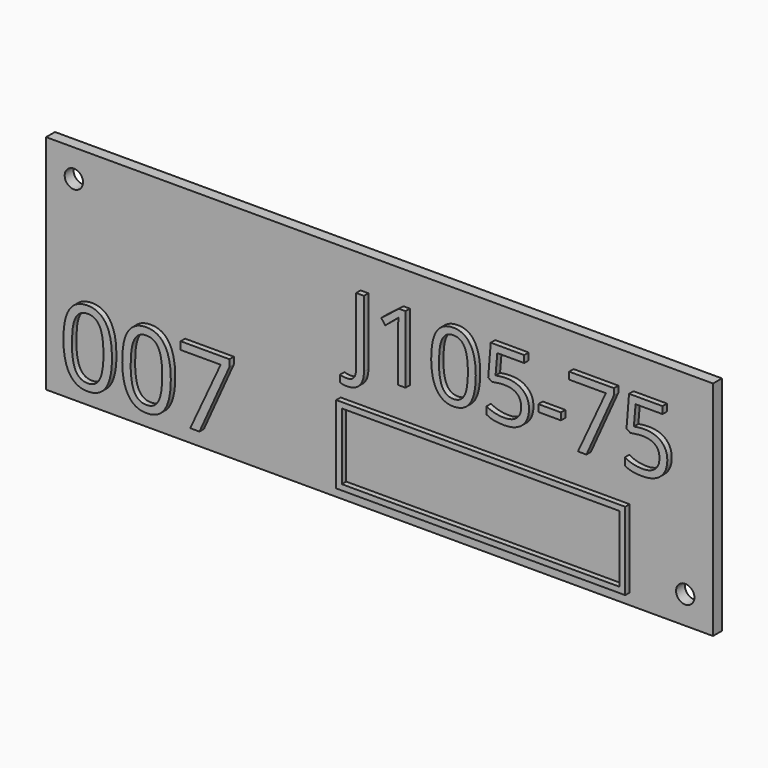
from build123d import *

# Parameters (mm, degrees)
F0_W         = 120
F0_H         = 40
F1_DEPTH     = 2
F3_D         = 3.3
F4_TEXT_SIZE = 16.9836355595
F5_DEPTH     = 1
F6_TEXT_SIZE = 18.5054667028
F7_DEPTH     = 1
F8_W         = 52
F8_H         = 14
F8_W_2       = 49.99999962
F8_H_2       = 11.99999962
F9_DEPTH     = 1


# Not quite as in the source:
# - Text() gives the source's letters only with a copy of the font that has no kerning and outlines rounded to 1/6400 em; it was checked with that copy


with BuildPart() as f1:
    # F0 (on Front) → F1 (new body)
    with BuildSketch(Plane.XZ):
        Rectangle(F0_W, F0_H)
    extrude(amount=F1_DEPTH)

    # F3 (through all)
    with Locations(Plane.XZ.offset(2)):
        with Locations((-55, 15), (55, -15)):
            Hole(F3_D / 2)

    # F4 (on face) → F5 (join)
    with BuildSketch(Plane.XZ.offset(2)):
        with Locations((-5, 2)):
            Text('J105-75', F4_TEXT_SIZE, font='Open Sans', text_align=(TextAlign.LEFT, TextAlign.BOTTOM))
    extrude(amount=F5_DEPTH)

    # F6 (on face) → F7 (join)
    with BuildSketch(Plane.XZ.offset(2)):
        with Locations((-57, -17)):
            Text('007', F6_TEXT_SIZE, font='Open Sans', text_align=(TextAlign.LEFT, TextAlign.BOTTOM))
    extrude(amount=F7_DEPTH)

    # F8 (on face) → F9 (join)
    with BuildSketch(Plane.XZ.offset(2)):
        with Locations((19, -11)):
            Rectangle(F8_W, F8_H)
        with Locations((19, -11)):
            Rectangle(F8_W_2, F8_H_2, mode=Mode.SUBTRACT)
    extrude(amount=F9_DEPTH)


solid = f1.part
